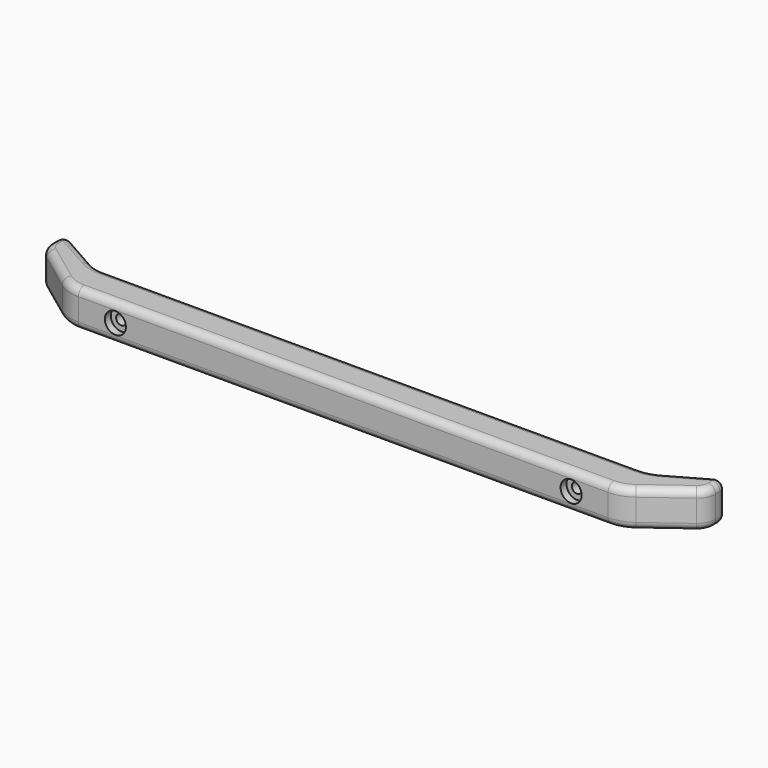
from build123d import *

# Parameters (mm, degrees)
F1_DEPTH = 10
F2_R     = 2
F3_R     = 1.4
F4_DEPTH = 11
F3_R_2   = 2.85
F5_DEPTH = 2


with BuildPart() as f1:
    # F0 (on Top) → F1 (new body)
    with BuildSketch(Plane.XY):
        with BuildLine():
            ThreePointArc((77.2961207269, 6.3033039919), (74.9125256302, 5.3313144616), (72.3597780987, 5))
            Line((72.3597780987, 5), (0, 5))
            Line((0, 5), (0, -5))
            Line((0, -5), (71.6958680115, -5))
            ThreePointArc((71.6958680115, -5), (74.8331804116, -4.495118267), (77.6536984673, -3.0314541808))
            Line((77.6536984673, -3.0314541808), (87.9106565848, 4.5772821801))
            ThreePointArc((87.9106565848, 4.5772821801), (89.3979800506, 6.3451854495), (89.9317413568, 8.5930092705))
            Line((89.9317413568, 8.5930092705), (89.9317413568, 10.0404781398))
            ThreePointArc((89.9317413568, 10.0404781398), (88.9380869607, 11.7688497797), (86.9444728312, 11.7798173414))
            Line((86.9444728312, 11.7798173414), (77.2961207269, 6.3033039919))
        make_face()
    extrude(amount=F1_DEPTH)

    # F2
    f2_edges = [f1.edges().sort_by_distance(p)[0] for p in [
        (35.847934, -5, 10),
        (35.847934, -5, 0),
    ]]
    fillet(f2_edges, radius=F2_R)

    # F3 (on face) → F4 (cut)
    with BuildSketch(Plane.XZ.offset(5)):
        with Locations((61.6958680115, 5)):
            Circle(F3_R)
    extrude(amount=-F4_DEPTH, mode=Mode.SUBTRACT)

    # F3 (on face) → F5 (cut)
    with BuildSketch(Plane.XZ.offset(5)):
        with Locations((61.6958680115, 5)):
            Circle(F3_R_2)
        with Locations((61.6958680115, 5)):
            Circle(F3_R, mode=Mode.SUBTRACT)
    extrude(amount=-F5_DEPTH, mode=Mode.SUBTRACT)

    # F6: F1 across plane


with BuildPart() as f1_1:
    add(f1.part)
    add(f1.part.mirror(Plane.YZ))


solid = f1_1.part
